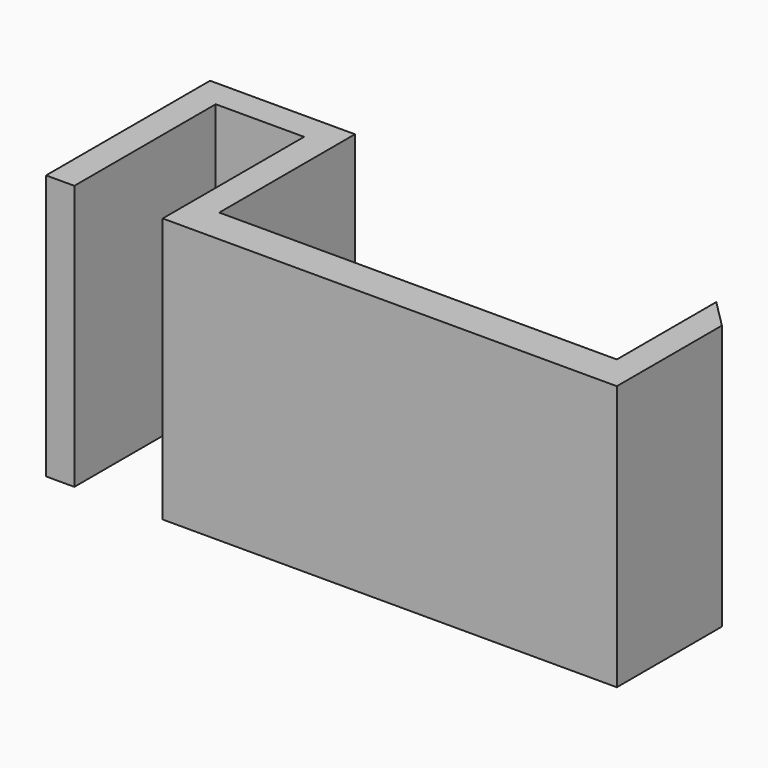
from build123d import *

# Parameters (mm, degrees)
F1_DEPTH    = 30
F2_T1_DEPTH = 55.7168298797


# Not quite as in the source:
# - a fillet or chamfer that OpenCascade refuses, or shapes differently, is made with other operations: its cross-section is extruded or revolved along the edge and cut away or added


with BuildPart() as f1:
    # F0 (on Top) → F1 (new body)
    with BuildSketch(Plane.XY):
        Polygon((-3.2, 0), (0, 0), (0, 20), (10, 20), (10, 0), (13.2, 0), (58.2, 0), (61.4, 0), (61.4, 19.8679156601), (58.2, 19.8679156601), (58.2, 4.00000019), (13.2, 4.00000019), (13.2, 23.2), (-3.2, 23.2), align=None)
    extrude(amount=F1_DEPTH)

    # F2: chamfer of 5 on 1 edges, made by hand

    # F2_s2 → F2_t1 (cut)
    with BuildSketch(Plane.XY.offset(-12.8584149398)):
        Polygon((56.4, 19.8679156601), (61.4, 14.8679156601), (61.4, 19.8679156601), align=None)
    extrude(amount=F2_T1_DEPTH, mode=Mode.SUBTRACT)


solid = f1.part
